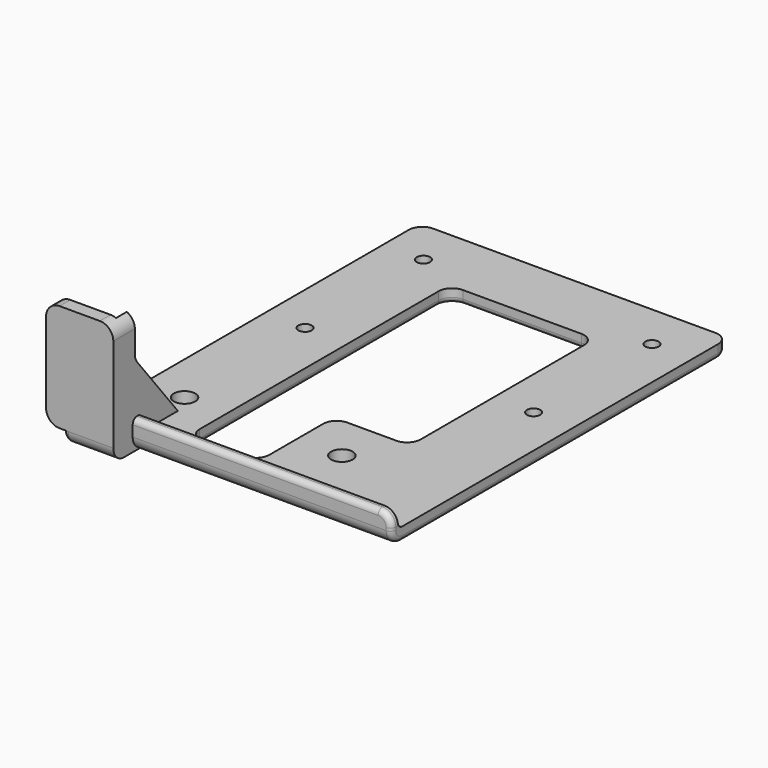
from build123d import *

# Parameters (mm, degrees)
F0_W      = 115
F0_H      = 165.8
F0_R      = 4
F0_R_2    = 2.5
F1_DEPTH  = 5
F2_W      = 18.7665516138
F2_H      = 5
F2_W_2    = 6.2334483862
F3_DEPTH  = 40
F4_W      = 3
F4_H      = 25
F5_DEPTH  = 25
F9_W      = 3
F9_H      = 5
F10_DEPTH = 14.58
F12_DEPTH = 3
F13_W     = 96.2334483862
F13_H     = 9
F14_DEPTH = 5
F15_W     = 96.2334483862
F15_H     = 3
F16_DEPTH = 6
F17_R     = 5
F18_R     = 2


with BuildPart() as f1:
    # F0 (on Top) → F1 (new body)
    with BuildSketch(Plane.XY):
        with Locations((-57.5, 82.9)):
            Rectangle(F0_W, F0_H)
        with Locations((-100, 37.8)):
            Circle(F0_R, mode=Mode.SUBTRACT)
        with Locations((-41.5, 37.8)):
            Circle(F0_R, mode=Mode.SUBTRACT)
        Polygon((-84.125764668, 141.0401467979), (-30, 141.0401467979), (-30, 55), (-58.2305043936, 55), (-58.2305043936, 20), (-84.125764668, 20), align=None, mode=Mode.SUBTRACT)
        with Locations((-100, 93.8)):
            Circle(F0_R_2, mode=Mode.SUBTRACT)
        with Locations((-100, 148.8)):
            Circle(F0_R_2, mode=Mode.SUBTRACT)
        with Locations((-15, 93.8)):
            Circle(F0_R_2, mode=Mode.SUBTRACT)
        with Locations((-15, 148.8)):
            Circle(F0_R_2, mode=Mode.SUBTRACT)
    extrude(amount=-F1_DEPTH)

    # F2 (on face) → F3 (join)
    with BuildSketch(Plane(origin=(0, 0, -5), x_dir=(1, 0, 0), z_dir=(0, 0, -1))):
        with Locations((-105.6167241931, -2.5)):
            Rectangle(F2_W, F2_H)
        with Locations((-118.1167241931, -2.5)):
            Rectangle(F2_W_2, F2_H)
    extrude(amount=F3_DEPTH)

    # F4 (on face) → F5 (join)
    with BuildSketch(Plane(origin=(0, 5, 0), x_dir=(-1, 0, 0), z_dir=(0, 1, 0))):
        with Locations((97.7334483862, -17.5)):
            Rectangle(F4_W, F4_H)
    extrude(amount=F5_DEPTH)


with BuildPart() as f7_1:
    # F7: instance of F1
    add(f1.part.mirror(Plane.XY))

    # F9 (on face) → F10 (join)
    with BuildSketch(Plane.XY.offset(30)):
        with Locations((-97.7334483862, 7.5)):
            Rectangle(F9_W, F9_H)
    extrude(amount=F10_DEPTH)

    # F11 (on face) → F12 (cut, through all)
    with BuildSketch(Plane(origin=(-99.2334483862, 0, 0), x_dir=(0, -1, 0), z_dir=(-1, 0, 0))):
        Polygon((-30, 30), (-30, 5), (-10, 30), align=None)
    extrude(amount=-F12_DEPTH, mode=Mode.SUBTRACT)

    # F13 (on face) → F14 (cut, through all)
    with BuildSketch(Plane.XY.offset(5)):
        with Locations((-48.1167241931, 4.5)):
            Rectangle(F13_W, F13_H)
    extrude(amount=-F14_DEPTH, mode=Mode.SUBTRACT)

    # F15 (on face) → F16 (join)
    with BuildSketch(Plane.XY.offset(5)):
        with Locations((-48.1167241931, 10.5)):
            Rectangle(F15_W, F15_H)
    extrude(amount=F16_DEPTH)

    # F17
    f17_edges = [f7_1.edges().sort_by_distance(p)[0] for p in [
        (-97.733448, 10, 30),
        (-105.616724, 0, 0),
        (-96.233448, 2.5, 45),
        (-121.233448, 2.5, 45),
        (-121.233448, 2.5, 5),
        (-115, 165.8, 2.5),
        (0, 165.8, 2.5),
        (0, 10.5, 11),
        (-58.230504, 55, 2.5),
        (-30, 55, 2.5),
        (-58.230504, 20, 2.5),
        (-84.125765, 20, 2.5),
        (-30, 141.040147, 2.5),
        (-84.125765, 141.040147, 2.5),
        (-48.116724, 9, 0),
    ]]
    fillet(f17_edges, radius=F17_R)

    # F18 (call 1 of 4: OpenCascade refuses the feature's edges together)
    f18_edges = [f7_1.edges().sort_by_distance(p)[0] for p in [
        (-48.116724, 12, 5),
    ]]
    fillet(f18_edges, radius=F18_R)

    # F18#2 (call 2 of 4)
    f18_2_edges = [f7_1.edges().sort_by_distance(p)[0] for p in [
        (-107.116724, 5, 5),
    ]]
    fillet(f18_2_edges, radius=F18_R)

    # F18#3 (call 3 of 4)
    f18_3_edges = [f7_1.edges().sort_by_distance(p)[0] for p in [
        (0, 87.4, 0),
        (-115, 1.464466, 1.464466),
        (-115, 82.9, 0),
        (-113.535534, 164.335534, 0),
        (-57.5, 165.8, 0),
        (-1.464466, 164.335534, 0),
        (-50.616724, 9, 11),
        (0, 9, 5.5),
        (-1.464466, 9, 9.535534),
        (0, 10.464466, 1.464466),
    ]]
    fillet(f18_3_edges, radius=F18_R)

    # F18#4 (call 4 of 4)
    f18_4_edges = [f7_1.edges().sort_by_distance(p)[0] for p in [
        (-30, 98.020073, 0),
        (-57.062882, 141.040147, 0),
        (-82.661299, 139.575681, 0),
        (-31.464466, 139.575681, 0),
        (-84.125765, 80.520073, 0),
        (-82.661299, 21.464466, 0),
        (-31.464466, 56.464466, 0),
        (-71.178135, 20, 0),
        (-44.115252, 55, 0),
        (-59.69497, 21.464466, 0),
        (-56.766038, 53.535534, 0),
        (-58.230504, 37.5, 0),
    ]]
    fillet(f18_4_edges, radius=F18_R)


solid = f7_1.part
